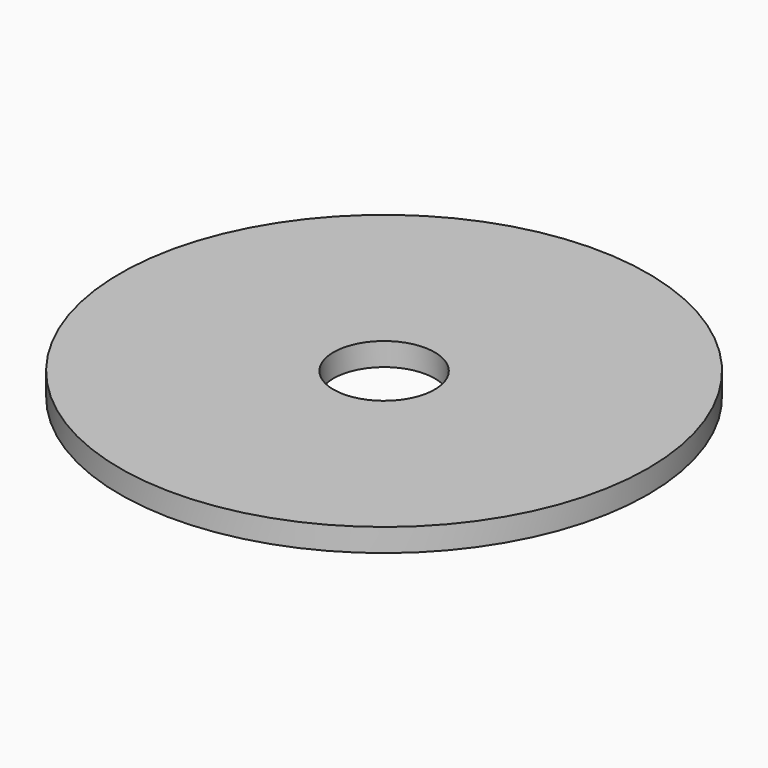
from build123d import *

# Parameters (mm, degrees)
F0_R     = 34.4457602684
F1_DEPTH = 3
F3_D     = 13.2


# Not quite as in the source:
# - a feature names something its author has since deleted; it is built from what else it names


with BuildPart() as f1:
    # F0 (on Top) → F1 (new body)
    with BuildSketch(Plane.XY):
        Circle(F0_R)
    extrude(amount=-F1_DEPTH)

    # F3 (through all)
    with Locations(Plane.XY):
        with Locations((0, 0)):
            Hole(F3_D / 2)


with BuildPart() as f4_1:
    # F4: copy of F1
    add(f1.part)


with BuildPart() as f6_1:
    # F6: copy of F1
    add(f1.part)


solid = Compound([f1.part, f6_1.part])
